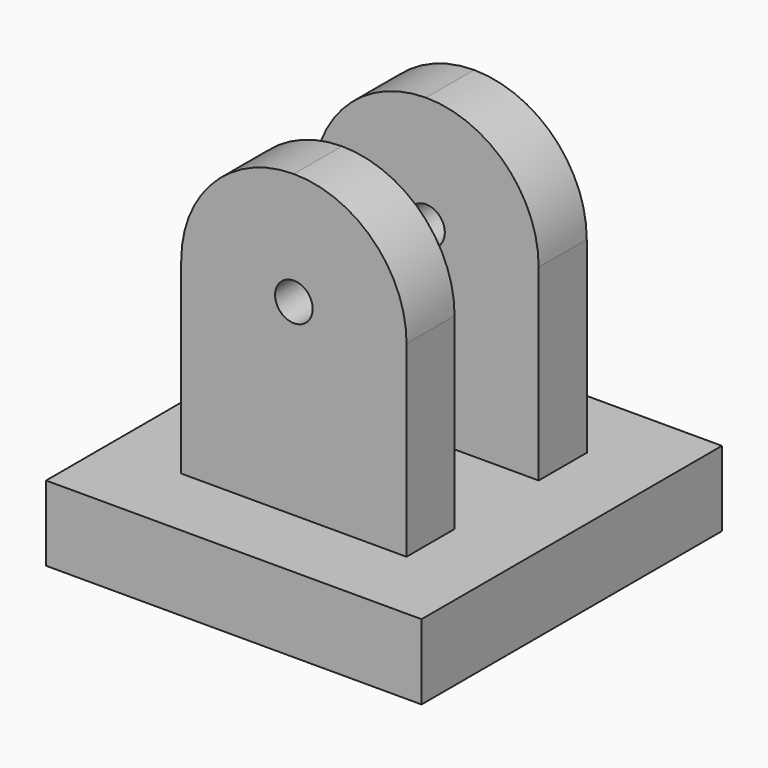
from build123d import *

# Parameters (mm, degrees)
F0_W     = 50
F0_H     = 50
F1_DEPTH = 10
F2_W     = 30
F2_H     = 8
F3_DEPTH = 50
F4_R     = 14.99999
F6_D     = 5


# Not quite as in the source:
# - a fillet or chamfer is up to 0.001 mm smaller than in the source, because OpenCascade refuses the exact size


with BuildPart() as f1:
    # F0 (on Top) → F1 (new body)
    with BuildSketch(Plane.XY):
        Rectangle(F0_W, F0_H)
    extrude(amount=F1_DEPTH)

    # F2 (on Top) → F3 (join)
    with BuildSketch(Plane.XY):
        with Locations((0, 11)):
            Rectangle(F2_W, F2_H)
        with Locations((0, -11)):
            Rectangle(F2_W, F2_H)
    extrude(amount=F3_DEPTH)

    # F4 (radius 15 in the source; OpenCascade refuses exactly that, so slightly less here)
    f4_edges = [f1.edges().sort_by_distance(p)[0] for p in [
        (-15, -11, 50),
        (-15, 11, 50),
        (15, 11, 50),
        (15, -11, 50),
    ]]
    fillet(f4_edges, radius=F4_R)

    # F6 (through all)
    with Locations(Plane.XZ.offset(15)):
        with Locations((0, 35)):
            Hole(F6_D / 2)


solid = f1.part
